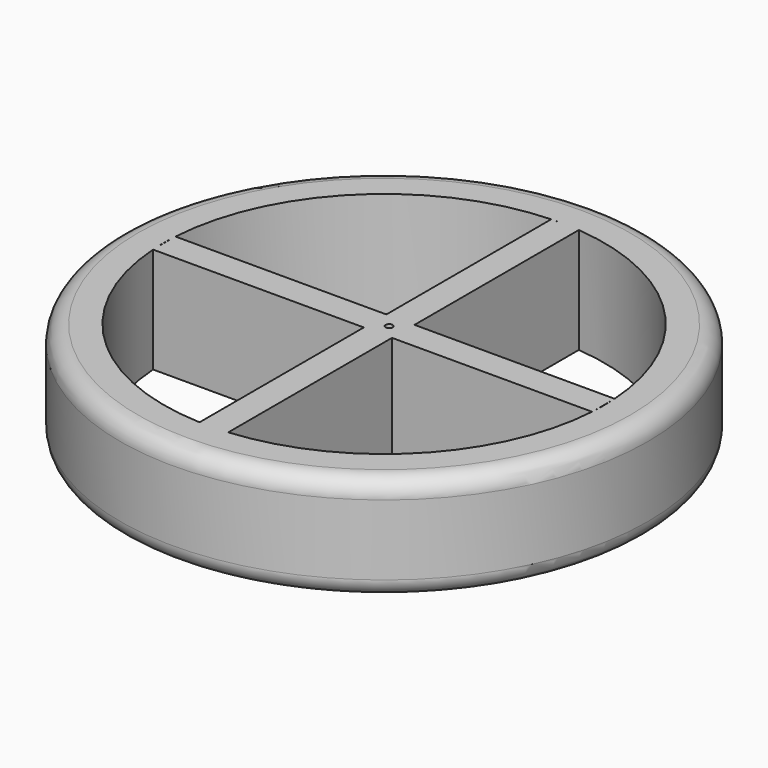
from build123d import *

# Parameters (mm, degrees)
F0_R      = 75
F1_DEPTH  = 30
F2_R      = 5
F3_R      = 5
F4_R      = 62.5
F5_DEPTH  = 30
F7_E2_W   = 124.9627603046
F7_E2_H   = 30
F8_DEPTH  = 4
F10_E3_W  = 124.8690485954
F10_E3_H  = 30
F11_DEPTH = 4
F12_R     = 1
F13_DEPTH = 12
F14_R     = 1
F15_DEPTH = 12


with BuildPart() as f1:
    # F0 (on Top) → F1 (new body)
    with BuildSketch(Plane.XY):
        with Locations((-35.8805991709, 25.7855858654)):
            Circle(F0_R)
    extrude(amount=F1_DEPTH)

    # F2
    f2_edges = [f1.edges().sort_by_distance(p)[0] for p in [
        (-110.880599, 25.785586, 0),
    ]]
    fillet(f2_edges, radius=F2_R)

    # F3
    f3_edges = [f1.edges().sort_by_distance(p)[0] for p in [
        (-110.880599, 25.785586, 30),
    ]]
    fillet(f3_edges, radius=F3_R)

    # F4 (on face) → F5 (cut)
    with BuildSketch(Plane(origin=(0, 0, 0), x_dir=(1, 0, 0), z_dir=(0, 0, -1))):
        with Locations((-35.8805991709, -25.7855858654)):
            Circle(F4_R)
    extrude(amount=-F5_DEPTH, mode=Mode.SUBTRACT)

    # F7_E2 (on explicit) → F8 (join, symmetric)
    with BuildSketch(Plane(origin=(-34.3551044097, 88.2669660177, 0), x_dir=(0, -1, 0), z_dir=(-1, 0, 0))):
        with Locations((62.4813801523, 15)):
            Rectangle(F7_E2_W, F7_E2_H)
    extrude(amount=F8_DEPTH, both=True)

    # F10_E3 (on explicit) → F11 (join, symmetric)
    with BuildSketch(Plane(origin=(-98.322533071, 25.6824456155, 0), x_dir=(1, 0, 0), z_dir=(0, -1, 0))):
        with Locations((62.4345242977, 15)):
            Rectangle(F10_E3_W, F10_E3_H)
    extrude(amount=F11_DEPTH, both=True)

    # F12 (on face) → F13 (cut)
    with BuildSketch(Plane.XY.offset(30)):
        with Locations((-34.3549661338, 25.6826244295)):
            Circle(F12_R)
    extrude(amount=-F13_DEPTH, mode=Mode.SUBTRACT)

    # F14 (on Top) → F15 (cut)
    with BuildSketch(Plane.XY):
        with Locations((-34.3551188707, 25.6825555116)):
            Circle(F14_R)
    extrude(amount=F15_DEPTH, mode=Mode.SUBTRACT)


solid = f1.part
